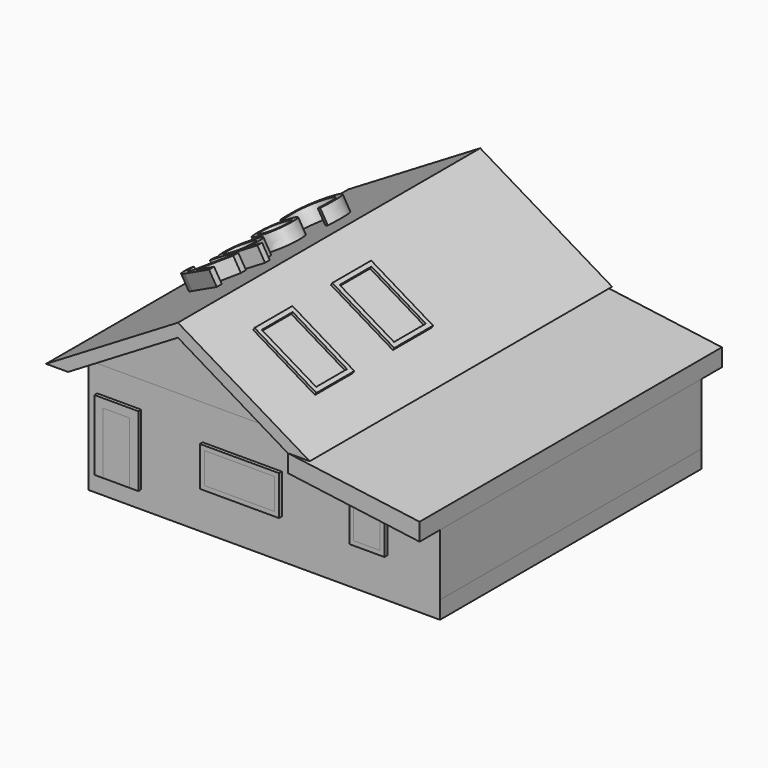
from build123d import *

# Parameters (mm, degrees)
F1_DEPTH      = 914.4
F1_DEPTH_BACK = 12192
F2_DEPTH      = 30.48
F2_DEPTH_BACK = 11277.6
F0_W          = 2743.2
F0_H          = 1371.6
F0_W_2        = 1219.2
F3_DEPTH      = 30.48
F3_DEPTH_BACK = 11277.6
F4_DEPTH      = 30.48
F4_DEPTH_BACK = 11277.6
F0_W_3        = 2438.4
F0_H_2        = 1066.8
F5_DEPTH      = 152.4
F5_DEPTH_BACK = 11277.6
F0_W_4        = 914.4
F0_H_3        = 2133.6
F6_DEPTH      = 152.4
F7_W          = 2133.6
F7_H          = 1371.6
F7_W_2        = 1828.8
F7_H_2        = 1066.8
F8_DEPTH      = 152.4
F9_W          = 2503.7041634834
F9_H          = 1643.1843989028
F9_W_2        = 2198.9041634834
F9_H_2        = 1338.3843989028
F9_H_3        = 1683.6252212524
F9_H_4        = 1378.8252212524
F10_DEPTH     = 91.44
F11_W         = 1219.2
F11_H         = 1371.6
F11_W_2       = 2743.2
F12_DEPTH     = 30.48
F13_TEXT_SIZE = 2523.5705045278
F14_DEPTH     = 518.16


# Not quite as in the source:
# - a feature names something its author has since deleted; it is built from what else it names
# - Text() gives the source's letters only with a copy of the font that has no kerning and outlines rounded to 1/6400 em; it was checked with that copy


with BuildPart() as f1:
    # F0 (on Front) → F1 (new body, two sides)
    with BuildSketch(Plane.XZ) as f1_sk:
        Polygon((8381.1556260289, -609.6), (3810, 0), (3810, -609.6), (8381.3432646803, -1219.1999711218), align=None)
    extrude(amount=F1_DEPTH)
    extrude(f1_sk.sketch, amount=-F1_DEPTH_BACK)



with BuildPart() as f1b:
    # F0 (on Front) → F1, piece 2 (new body, two sides)
    with BuildSketch(Plane.XZ) as f1_2_sk:
        Polygon((0, 2286), (3810, 0), (4572, 0), (0, 2743.2), align=None)
        Polygon((-4572, 0), (-3810, 0), (0, 2286), (0, 2743.2), align=None)
    extrude(amount=F1_DEPTH)
    extrude(f1_2_sk.sketch, amount=-F1_DEPTH_BACK)


with BuildPart() as f1_1:
    add(f1.part)

    add(f1b.part)  # F2 merges F1b
    # F0 (on Front) → F2 (join, two sides)
    with BuildSketch(Plane.XZ) as f2_sk:
        Polygon((-3810, 0), (0, 0), (0, 2286), align=None)
        Polygon((0, 2286), (0, 0), (3810, 0), align=None)
    extrude(amount=F2_DEPTH)
    extrude(f2_sk.sketch, amount=-F2_DEPTH_BACK)

    # F9 (on face) → F10 (join)
    with BuildSketch(Plane(origin=(1210.2352941176, 0, 2017.0588235294), x_dir=(0.8574929257, 0, -0.5144957554), z_dir=(0.5144957554, 0, 0.8574929257))):
        with Locations((1099.4520817417, 1819.5399784073)):
            Rectangle(F9_W, F9_H)
        with Locations((1099.4520817417, 1819.5399784073)):
            Rectangle(F9_W_2, F9_H_2, mode=Mode.SUBTRACT)
        with Locations((1099.4520817417, 5213.695526123)):
            Rectangle(F9_W, F9_H_3)
        with Locations((1099.4520817417, 5213.695526123)):
            Rectangle(F9_W_2, F9_H_4, mode=Mode.SUBTRACT)
    extrude(amount=F10_DEPTH)

    # F13 (on face) → F14 (join)
    with BuildSketch(Plane(origin=(-1210.2352941176, 0, 2017.0588235294), x_dir=(0.8574929257, 0, 0.5144957554), z_dir=(-0.5144957554, 0, 0.8574929257))):
        with Locations(Location((-1969.8596420768, 8877.4775611808), (0, 0, -90))):
            Text('Cody', F13_TEXT_SIZE, font='Open Sans', text_align=(TextAlign.LEFT, TextAlign.BOTTOM))
    extrude(amount=F14_DEPTH)


with BuildPart() as f3:
    # F0 (on Front) → F3 (new body, two sides)
    with BuildSketch(Plane.XZ) as f3_sk:
        Polygon((3810, 0), (0, 0), (-3810, 0), (-3810, -3352.8), (-3505.2, -3352.8), (-3505.2, -914.4), (-1981.2, -914.4), (-1981.2, -3352.8), (3810, -3352.8), (3810, -609.6), align=None)
        with Locations((1524, -1905)):
            Rectangle(F0_W, F0_H, mode=Mode.SUBTRACT)
        Polygon((8381.3432646803, -1219.1999711218), (3810, -609.6), (3810, -3352.8), (8382, -3352.8), align=None)
        with Locations((5943.6, -1905)):
            Rectangle(F0_W_2, F0_H, mode=Mode.SUBTRACT)
    extrude(amount=F3_DEPTH)
    extrude(f3_sk.sketch, amount=-F3_DEPTH_BACK)

    # F0 (on Front) → F4 (join, two sides)
    with BuildSketch(Plane.XZ) as f4_sk:
        Polygon((-3505.2, -3352.8), (-3810, -3352.8), (-3810, -3962.4), (3810, -3962.4), (8382, -3962.4), (8382, -3352.8), (3810, -3352.8), (-1981.2, -3352.8), (-2286, -3352.8), (-3200.4, -3352.8), align=None)
    extrude(amount=F4_DEPTH)
    extrude(f4_sk.sketch, amount=-F4_DEPTH_BACK)

    # F0 (on Front) → F5, piece 2 (join, two sides)
    with BuildSketch(Plane.XZ) as f5_2_sk:
        with Locations((-2743.2, -2286)):
            Rectangle(F0_W_4, F0_H_3)
    extrude(amount=F5_DEPTH)
    extrude(f5_2_sk.sketch, amount=-F5_DEPTH_BACK)

    # F7 (on face) → F8 (join)
    with BuildSketch(Plane(origin=(-3810, 0, 0), x_dir=(0, -1, 0), z_dir=(-1, 0, 0))):
        with Locations((-8498.0065870829, -2289.1992926598)):
            Rectangle(F7_W, F7_H)
        with Locations((-8498.0065870829, -2289.1992926598)):
            Rectangle(F7_W_2, F7_H_2, mode=Mode.SUBTRACT)
        with Locations((-4187.9855377197, -2289.1992926598)):
            Rectangle(F7_W, F7_H)
        with Locations((-4187.9855377197, -2289.1992926598)):
            Rectangle(F7_W_2, F7_H_2, mode=Mode.SUBTRACT)
    extrude(amount=F8_DEPTH)


with BuildPart() as f5:
    # F0 (on Front) → F5 (new body, two sides)
    with BuildSketch(Plane.XZ) as f5_sk:
        with Locations((1524, -1905)):
            Rectangle(F0_W_3, F0_H_2)
    extrude(amount=F5_DEPTH)
    extrude(f5_sk.sketch, amount=-F5_DEPTH_BACK)


with BuildPart() as f5b:
    # F0 (on Front) → F5, piece 3 (new body, two sides)
    with BuildSketch(Plane.XZ) as f5_3_sk:
        with Locations((5943.6, -1905)):
            Rectangle(F0_W_4, F0_H_2)
    extrude(amount=F5_DEPTH)
    extrude(f5_3_sk.sketch, amount=-F5_DEPTH_BACK)


with BuildPart() as f6:
    # F0 (on Front) → F6 (new body)
    with BuildSketch(Plane.XZ):
        with Locations((5943.6, -1905)):
            Rectangle(F0_W_2, F0_H)
        with Locations((5943.6, -1905)):
            Rectangle(F0_W_4, F0_H_2, mode=Mode.SUBTRACT)
    extrude(amount=F6_DEPTH)


with BuildPart() as f6b:
    # F0 (on Front) → F6, piece 2 (new body)
    with BuildSketch(Plane.XZ):
        Polygon((-3505.2, -914.4), (-3505.2, -3352.8), (-3200.4, -3352.8), (-3200.4, -1219.2), (-2286, -1219.2), (-2286, -3352.8), (-1981.2, -3352.8), (-1981.2, -914.4), align=None)
    extrude(amount=F6_DEPTH)


with BuildPart() as f6c:
    # F0 (on Front) → F6, piece 3 (new body)
    with BuildSketch(Plane.XZ):
        with Locations((1524, -1905)):
            Rectangle(F0_W, F0_H)
        with Locations((1524, -1905)):
            Rectangle(F0_W_3, F0_H_2, mode=Mode.SUBTRACT)
    extrude(amount=F6_DEPTH)


with BuildPart() as f12:
    # F11 (on face) → F12 (new body)
    with BuildSketch(Plane(origin=(0, 11277.6, 0), x_dir=(-1, 0, 0), z_dir=(0, 1, 0))):
        Polygon((3810, -3962.4), (3810, 0), (-3810, 0), (-3810, -609.6), (-8381.3432646803, -1219.1999711218), (-8382, -3352.8), (-8382, -3962.4), align=None)
        Polygon((1981.2, -914.4), (3505.2, -914.4), (3505.2, -3352.8), (3200.4, -3352.8), (3200.4, -1219.2), (2286, -1219.2), (2286, -3352.8), (1981.2, -3352.8), align=None, mode=Mode.SUBTRACT)
        with Locations((-5943.6, -1905)):
            Rectangle(F11_W, F11_H, mode=Mode.SUBTRACT)
        with Locations((-1524, -1905)):
            Rectangle(F11_W_2, F11_H, mode=Mode.SUBTRACT)
        with Locations((-1524, -1905)):
            Rectangle(F11_W_2, F11_H)
    extrude(amount=F12_DEPTH)


solid = Compound([f1_1.part, f3.part, f5.part, f5b.part, f6.part, f6b.part, f6c.part, f12.part])
